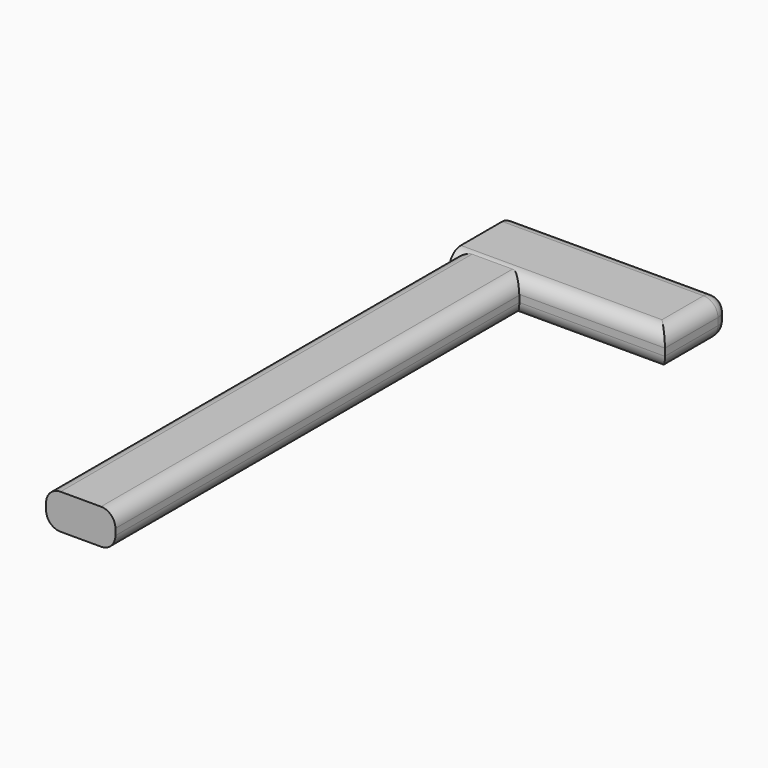
from build123d import *

# Parameters (mm, degrees)
F0_W         = 75.9326070547
F0_H         = 28.4124165773
F1_DEPTH     = 12.7
F2_W         = 24.4196355343
F2_H         = 12.4133229256
F3_DEPTH     = 177.8
F4_T1_DEPTH  = 53.8124165773
F4_T3_DEPTH  = 63.9811988592
F4_T5_DEPTH  = 190.5
F4_T10_DEPTH = 101.3326070547
F4_T16_DEPTH = 101.3326070547
F4_T22_DEPTH = 101.3326070547
F4_T29_DEPTH = 101.3326070547
F4_T35_DEPTH = 101.3326070547
F4_T42_DEPTH = 76.6811988592
F4_T46_DEPTH = 203.2
F5_R         = 5.08
F6_R         = 5.08


# Not quite as in the source:
# - a fillet or chamfer that OpenCascade refuses, or shapes differently, is made with other operations: its cross-section is extruded or revolved along the edge and cut away or added


with BuildPart() as f1:
    # F0 (on Top) → F1 (new body)
    with BuildSketch(Plane.XY):
        with Locations((-37.9663035274, 14.2062082887)):
            Rectangle(F0_W, F0_H)
    extrude(amount=F1_DEPTH)

    # F2 (on Front) → F3 (join)
    with BuildSketch(Plane.XZ):
        with Locations((-63.4910166264, 6.2066614628)):
            Rectangle(F2_W, F2_H)
    extrude(amount=F3_DEPTH)

    # F4: fillet of radius 5.08 on 5 edges, made by hand

    # F4_s2 → F4_t1 (cut)
    with BuildSketch(Plane.XZ.offset(-41.1124165773)):
        with BuildLine():
            ThreePointArc((-5.08, 0), (-1.4878975516, 1.4878975516), (0, 5.08))
            Line((0, 5.08), (0, 0))
            Line((0, 0), (-5.08, 0))
        make_face()
        with BuildLine():
            ThreePointArc((0, 7.62), (-1.4878975516, 11.2121024484), (-5.08, 12.7))
            Line((-5.08, 12.7), (0, 12.7))
            Line((0, 12.7), (0, 7.62))
        make_face()
    extrude(amount=F4_T1_DEPTH, mode=Mode.SUBTRACT)

    # F4_s4 → F4_t3 (cut)
    with BuildSketch(Plane.YZ.offset(-51.2811988592)):
        with BuildLine():
            ThreePointArc((0, 5.08), (1.4878975516, 1.4878975516), (5.08, 0))
            Line((5.08, 0), (0, 0))
            Line((0, 0), (0, 5.08))
        make_face()
    extrude(amount=F4_T3_DEPTH, mode=Mode.SUBTRACT)

    # F4_s6 → F4_t5 (cut)
    with BuildSketch(Plane.XZ):
        with BuildLine():
            ThreePointArc((-56.3611988592, 0), (-52.7690964108, 1.4878975516), (-51.2811988592, 5.08))
            Line((-51.2811988592, 5.08), (-51.2811988592, 0))
            Line((-51.2811988592, 0), (-56.3611988592, 0))
        make_face()
    extrude(amount=F4_T5_DEPTH, mode=Mode.SUBTRACT)


with BuildPart() as f4_tool8:
    # F4_s9 → F4_t10 (new body)
    with BuildSketch(Plane.YZ.offset(-88.6326070547)):
        with BuildLine():
            ThreePointArc((0, 7.62), (1.4878975516, 11.2121024484), (5.08, 12.7))
            Line((5.08, 12.7), (0, 12.7))
            Line((0, 12.7), (0, 7.62))
        make_face()
    extrude(amount=F4_T10_DEPTH)

    split(bisect_by=Plane.YZ.offset(-75.7008343935), keep=Keep.BOTTOM)

    split(bisect_by=Plane.XY.offset(12.4133229256), keep=Keep.BOTTOM)


with BuildPart() as f1_1:
    add(f1.part)

    # F4_t7: cut F4_tool8
    add(f4_tool8.part, mode=Mode.SUBTRACT)


with BuildPart() as f4_tool14:
    # F4_s15 → F4_t16 (new body)
    with BuildSketch(Plane.YZ.offset(-88.6326070547)):
        with BuildLine():
            ThreePointArc((0, 7.62), (1.4878975516, 11.2121024484), (5.08, 12.7))
            Line((5.08, 12.7), (0, 12.7))
            Line((0, 12.7), (0, 7.62))
        make_face()
    extrude(amount=F4_T16_DEPTH)

    split(bisect_by=Plane.YZ.offset(-75.7008343935), keep=Keep.BOTTOM)

    split(bisect_by=Plane.XY.offset(12.4133229256), keep=Keep.TOP)


with BuildPart() as f1_2:
    add(f1_1.part)

    # F4_t13: cut F4_tool14
    add(f4_tool14.part, mode=Mode.SUBTRACT)


with BuildPart() as f4_tool20:
    # F4_s21 → F4_t22 (new body)
    with BuildSketch(Plane.YZ.offset(-88.6326070547)):
        with BuildLine():
            ThreePointArc((0, 7.62), (1.4878975516, 11.2121024484), (5.08, 12.7))
            Line((5.08, 12.7), (0, 12.7))
            Line((0, 12.7), (0, 7.62))
        make_face()
    extrude(amount=F4_T22_DEPTH)

    split(bisect_by=Plane.YZ.offset(-75.7008343935), keep=Keep.TOP)

    split(bisect_by=Plane.XY.offset(12.4133229256), keep=Keep.TOP)

    split(bisect_by=Plane.YZ.offset(-51.2811988592), keep=Keep.BOTTOM)


with BuildPart() as f1_3:
    add(f1_2.part)

    # F4_t19: cut F4_tool20
    add(f4_tool20.part, mode=Mode.SUBTRACT)


with BuildPart() as f4_tool27:
    # F4_s28 → F4_t29 (new body)
    with BuildSketch(Plane.YZ.offset(-88.6326070547)):
        with BuildLine():
            ThreePointArc((0, 7.62), (1.4878975516, 11.2121024484), (5.08, 12.7))
            Line((5.08, 12.7), (0, 12.7))
            Line((0, 12.7), (0, 7.62))
        make_face()
    extrude(amount=F4_T29_DEPTH)

    split(bisect_by=Plane.XY.offset(12.4133229256), keep=Keep.BOTTOM)

    split(bisect_by=Plane.YZ.offset(-51.2811988592), keep=Keep.TOP)


with BuildPart() as f1_4:
    add(f1_3.part)

    # F4_t26: cut F4_tool27
    add(f4_tool27.part, mode=Mode.SUBTRACT)


with BuildPart() as f4_tool33:
    # F4_s34 → F4_t35 (new body)
    with BuildSketch(Plane.YZ.offset(-88.6326070547)):
        with BuildLine():
            ThreePointArc((0, 7.62), (1.4878975516, 11.2121024484), (5.08, 12.7))
            Line((5.08, 12.7), (0, 12.7))
            Line((0, 12.7), (0, 7.62))
        make_face()
    extrude(amount=F4_T35_DEPTH)

    split(bisect_by=Plane.XY.offset(12.4133229256), keep=Keep.TOP)

    split(bisect_by=Plane.YZ.offset(-51.2811988592), keep=Keep.TOP)


with BuildPart() as f1_5:
    add(f1_4.part)

    # F4_t32: cut F4_tool33
    add(f4_tool33.part, mode=Mode.SUBTRACT)


with BuildPart() as f4_tool40:
    # F4_s41 → F4_t42 (new body)
    with BuildSketch(Plane.YZ.offset(-63.9811988592)):
        with BuildLine():
            ThreePointArc((0, 5.08), (1.4878975516, 1.4878975516), (5.08, 0))
            Line((5.08, 0), (0, 0))
            Line((0, 0), (0, 5.08))
        make_face()
    extrude(amount=F4_T42_DEPTH)

    split(bisect_by=Plane.YZ.offset(-51.2811988592), keep=Keep.BOTTOM)


with BuildPart() as f4_tool44:
    # F4_s45 → F4_t46 (new body)
    with BuildSketch(Plane.XZ.offset(-12.7)):
        with BuildLine():
            ThreePointArc((-56.3611988592, 0), (-52.7690964108, 1.4878975516), (-51.2811988592, 5.08))
            Line((-51.2811988592, 5.08), (-51.2811988592, 0))
            Line((-51.2811988592, 0), (-56.3611988592, 0))
        make_face()
    extrude(amount=F4_T46_DEPTH)

    split(bisect_by=Plane.XZ, keep=Keep.BOTTOM)


with BuildPart() as f4_tool40_1:
    add(f4_tool40.part)

    # F4_t48: intersect F4_tool44
    add(f4_tool44.part, mode=Mode.INTERSECT)


with BuildPart() as f1_6:
    add(f1_5.part)

    # F4_t38: cut F4_tool40
    add(f4_tool40_1.part, mode=Mode.SUBTRACT)

    # F5
    f5_edges = [f1_6.edges().sort_by_distance(p)[0] for p in [
        (-51.281199, -87.201198, 12.413323),
        (-75.700834, -87.201198, 12.413323),
        (-75.700834, -88.9, 0),
    ]]
    fillet(f5_edges, radius=F5_R)

    # F6
    f6_edges = [f1_6.edges().sort_by_distance(p)[0] for p in [
        (-75.932607, 14.206208, 0),
        (-75.932607, 28.412417, 6.35),
        (-40.506304, 28.412417, 0),
    ]]
    fillet(f6_edges, radius=F6_R)


solid = f1_6.part
